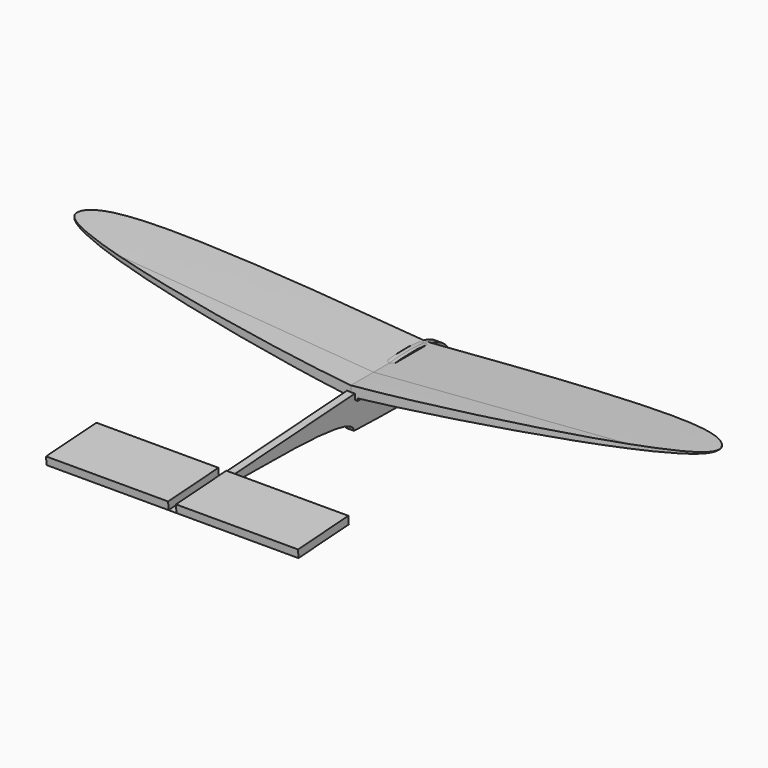
from build123d import *

# Parameters (mm, degrees)
F2_DEPTH = 65.786
F4_DEPTH = 3.175
F6_DEPTH = 63.5
F7_W     = 98.425
F7_H     = 50.8
F8_DEPTH = 6.35


with BuildPart() as f2:
    # F1 (on offset) → F2 (new body)
    with BuildSketch(Plane.XY.offset(21.59)):
        with BuildLine():
            add(Edge.make_bspline(
                [(0, 53.4413578779), (67.4104055153, 53.4586972971), (176.5463915152, 53.5165467261), (256.6457685576, 40.1454421025), (266.4896872291, -1.3911033325), (64.7221729159, -21.7577349395), (0, -22.9616686702)],
                knots=[0, 0, 0, 0, 0.3252822849, 0.5236438804, 0.6187167484, 1, 1, 1, 1], degree=3))
            add(Edge.make_bspline(
                [(0, 53.4413578779), (-67.4104055153, 53.4586972971), (-176.5463915152, 53.5165467261), (-256.6457685576, 40.1454421025), (-266.4896872291, -1.3911033325), (-64.7221729159, -21.7577349395), (0, -22.9616686702)],
                knots=[0, 0, 0, 0, 0.3252822849, 0.5236438804, 0.6187167484, 1, 1, 1, 1], degree=3))
        make_face()
    extrude(amount=F2_DEPTH)

    # F5 (on Front) → F6 (cut, symmetric)
    with BuildSketch(Plane.XZ):
        with BuildLine():
            Line((-5.1859715022, 18.8654828817), (-5.4291863926, 23.4526097775))
            add(Edge.make_bspline(
                [(-5.4291863926, 23.4526097775), (-132.3915962886, 36.1495305266), (-387.4886689374, 61.6606035868), (-129.557981055, 41.2534021875), (0, 31.0029126704)],
                knots=[0, 0, 0, 0, 0.4977023397, 1, 1, 1, 1], degree=3))
            add(Edge.make_bspline(
                [(5.4291863926, 23.4526097775), (132.3915962886, 36.1495305266), (387.4886689374, 61.6606035868), (129.557981055, 41.2534021875), (0, 31.0029126704)],
                knots=[0, 0, 0, 0, 0.4977023397, 1, 1, 1, 1], degree=3))
            Line((5.4291863926, 23.4526097775), (5.4291863926, 18.8654828817))
            Line((5.4291863926, 18.8654828817), (265.7273411751, 14.5721687004))
            Line((265.7273411751, 14.5721687004), (266.1809027195, 95.8389118314))
            Line((266.1809027195, 95.8389118314), (-269.0073251724, 95.8389118314))
            Line((-269.0073251724, 95.8389118314), (-265.6406164169, 15.9494355321))
            Line((-265.6406164169, 15.9494355321), (-5.1859715022, 18.8654828817))
        make_face()
    extrude(amount=F6_DEPTH, both=True, mode=Mode.SUBTRACT)


with BuildPart() as f4:
    # F3 (on Right) → F4 (new body, symmetric)
    with BuildSketch(Plane.YZ):
        with BuildLine():
            add(Edge.make_bspline(
                [(-23.4615208425, 26.1299874806), (10.8050309958, 31.1669088093), (67.8586209757, 39.4165856747), (80.7373193636, -6.2524051122), (13.9283636718, -0.5159713029), (-23.6930503499, 0)],
                knots=[0, 0, 0, 0, 0.4001961421, 0.5876085055, 1, 1, 1, 1], degree=3))
            Line((-23.4615208425, 26.1299874806), (-23.6930503499, 0))
        make_face()
        with BuildLine():
            Line((-23.6930503499, 0), (-23.4615208425, 26.1299874806))
            Line((-23.4615208425, 26.1299874806), (-202.6958614588, 14.4266597927))
            add(Edge.make_bspline(
                [(-202.6958614588, 14.4266597927), (-142.8293654074, 9.6177731951), (-24.6932628554, 17.6238827407), (-23.6930503499, 0)],
                knots=[0, 0, 0, 0, 179.5832255464, 179.5832255464, 179.5832255464, 179.5832255464], degree=3))
        make_face()
    extrude(amount=F4_DEPTH, both=True)


with BuildPart() as f8:
    # F7 (on face) → F8 (new body)
    with BuildSketch(Plane(origin=(0, -1.7985520105, 27.5444977919), x_dir=(1, 0, 0), z_dir=(0, -0.0651574804, 0.9978749935))):
        with Locations((52.3875, -175.9251266418)):
            Rectangle(F7_W, F7_H)
    extrude(amount=F8_DEPTH)


with BuildPart() as f8b:
    # F7 (on face) → F8, piece 2 (new body)
    with BuildSketch(Plane(origin=(0, -1.7985520105, 27.5444977919), x_dir=(1, 0, 0), z_dir=(0, -0.0651574804, 0.9978749935))):
        with Locations((-52.3875, -175.9251266418)):
            Rectangle(F7_W, F7_H)
    extrude(amount=F8_DEPTH)


solid = Compound([f2.part, f4.part, f8.part, f8b.part])
